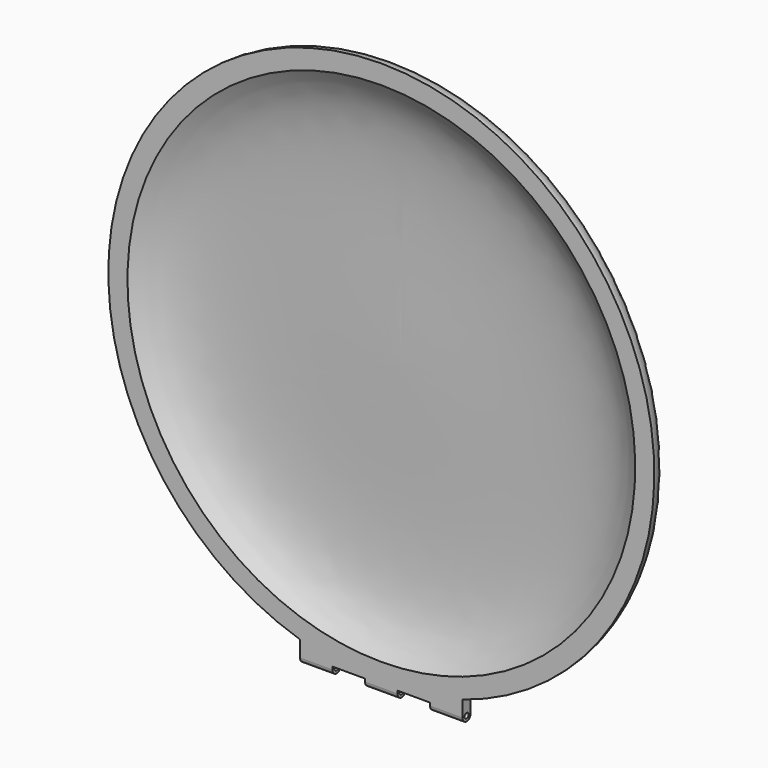
from build123d import *

# Parameters (mm, degrees)
F3_DEPTH = 1.27
F4_R     = 0.3175
F5_DEPTH = 44.2986001


# Not quite as in the source:
# - the dataset's text gives a spline's control points without its knots; the knots are read off the source's solid


with BuildPart() as f1:
    # F0 (on Right) → F1 (revolve)
    with BuildSketch(Plane.YZ):
        with BuildLine():
            add(Edge.make_bspline(
                [(3.175, 0), (3.175, 10.541), (4.0239762357, 25.9589322905), (0.7943624519, 30.4792560231), (0, 31.75)],
                knots=[0, 0, 0, 0, 0.6813666235, 1, 1, 1, 1], degree=3))
            Line((3.175, 0), (5.5626, 0))
            add(Edge.make_bspline(
                [(5.5626, 0), (5.5626, 1.9177725401), (5.6012595175, 5.763256361), (5.6850380944, 11.3740945743), (5.7026900101, 16.6481342132), (5.5838020802, 20.622627977), (5.3557319657, 23.480741035), (5.1437190397, 25.1246883423), (4.9215103036, 26.3507670581), (4.7229256392, 27.2307815663), (4.4932831777, 28.052608441), (4.1541081797, 29.0674517161), (3.6792176979, 30.1931579589), (2.8749355371, 31.7097687785), (2.3121014901, 32.5556376731), (2.0245751497, 33.015594415)],
                knots=[0, 0, 0, 0, 0.1249999999, 0.2499999998, 0.3749999996, 0.4999999995, 0.5624999995, 0.6249999994, 0.6562499994, 0.6874999993, 0.7187499993, 0.7499999993, 0.8124999992, 0.8749999991, 0.999999999, 0.999999999, 0.999999999, 0.999999999], degree=3))
            ThreePointArc((2.0245751497, 33.015594415), (1.1573462176, 33.8383446776), (0, 34.1376))
            Line((0, 34.1376), (0, 31.75))
        make_face()
    revolve(axis=Axis((0, 4.3688, 0), (0, 1, 0)))

    # F2 (on face) → F3 (join)
    with BuildSketch(Plane.XZ):
        with BuildLine():
            ThreePointArc((10.16, -30.0805069771), (0, -31.75), (-10.16, -30.0805069771))
            Line((-10.16, -30.0805069771), (-10.16, -35.2621069771))
            Line((-10.16, -35.2621069771), (-6.096, -35.2621069771))
            Line((-6.096, -35.2621069771), (-6.096, -34.2461069771))
            Line((-6.096, -34.2461069771), (-2.032, -34.2461069771))
            Line((-2.032, -34.2461069771), (-2.032, -35.2621069771))
            Line((-2.032, -35.2621069771), (2.032, -35.2621069771))
            Line((2.032, -35.2621069771), (2.032, -34.2461069771))
            Line((2.032, -34.2461069771), (6.096, -34.2461069771))
            Line((6.096, -34.2461069771), (6.096, -35.2621069771))
            Line((6.096, -35.2621069771), (10.16, -35.2621069771))
            Line((10.16, -35.2621069771), (10.16, -30.0805069771))
        make_face()
    extrude(amount=-F3_DEPTH)

    # F4 (on face) → F5 (cut, through all)
    with BuildSketch(Plane.YZ.offset(10.16)):
        with Locations((0.635, -34.622644881)):
            Circle(F4_R)
        with BuildLine():
            ThreePointArc((1.27, -34.622644881), (0.635, -35.257644881), (0, -34.622644881))
            Line((0, -34.622644881), (0, -35.2621069771))
            Line((0, -35.2621069771), (1.27, -35.2621069771))
            Line((1.27, -35.2621069771), (1.27, -34.622644881))
        make_face()
    extrude(amount=-F5_DEPTH, mode=Mode.SUBTRACT)


solid = f1.part
